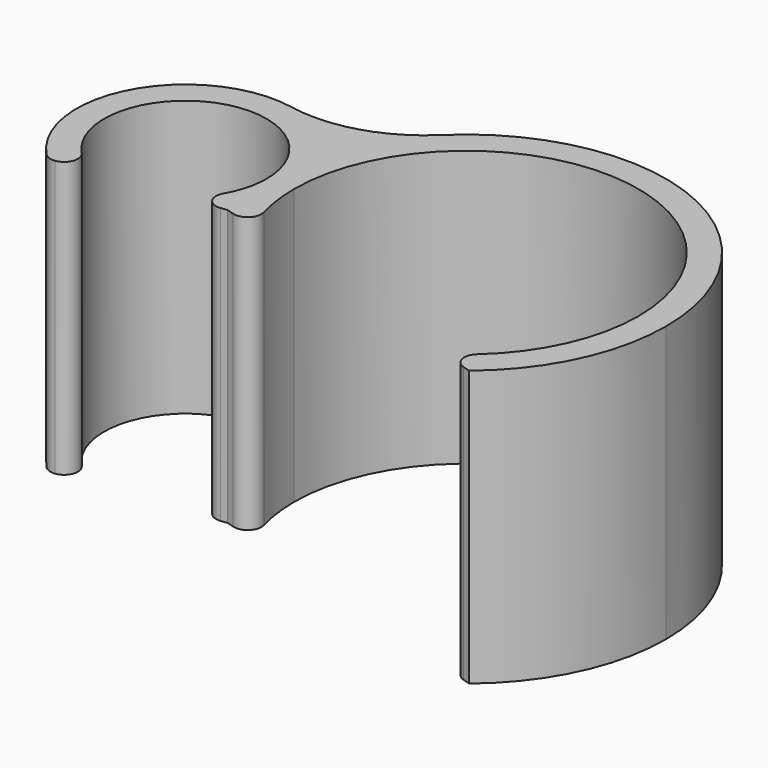
from build123d import *

# Parameters (mm, degrees)
F1_DEPTH = 10
F2_R     = 5
F3_R     = 0.49999


# Not quite as in the source:
# - a fillet or chamfer is up to 0.001 mm smaller than in the source, because OpenCascade refuses the exact size


with BuildPart() as f1:
    # F0 (on Top) → F1 (new body)
    with BuildSketch(Plane.XY):
        with BuildLine():
            ThreePointArc((-1.1283685941, -2.7256713514), (-1.6391785515, 2.4526707232), (2.95, 0))
            ThreePointArc((2.95, 0), (3.035057777, 1.107295327), (3.2882352941, 2.1886088391))
            ThreePointArc((3.2882352941, 2.1886088391), (-2.5695330315, 3), (-2.6678904245, -2.9128784188))
            Line((-2.6678904245, -2.9128784188), (-1.1283685941, -2.7256713514))
        make_face()
        with BuildLine():
            ThreePointArc((3.2882352941, 2.1886088391), (3.035057777, 1.107295327), (2.95, 0))
            ThreePointArc((2.95, 0), (3.035057777, -1.107295327), (3.2882352941, -2.1886088391))
            ThreePointArc((3.2882352941, -2.1886088391), (3.7809409815, -1.1432345753), (3.95, 0))
            ThreePointArc((3.95, 0), (3.7809409815, 1.1432345753), (3.2882352941, 2.1886088391))
        make_face()
        with BuildLine():
            ThreePointArc((3.2882352941, -2.1886088391), (3.035057777, -1.107295327), (2.95, 0))
            ThreePointArc((2.95, 0), (2.6326037224, -1.3311264557), (1.7487134637, -2.3758159065))
            Line((1.7487134637, -2.3758159065), (3.2882352941, -2.1886088391))
        make_face()
        with BuildLine():
            ThreePointArc((3.95, 0), (3.7809409815, -1.1432345753), (3.2882352941, -2.1886088391))
            Line((3.2882352941, -2.1886088391), (4.4925851142, -2.5471386536))
            ThreePointArc((4.4925851142, -2.5471386536), (4.0871511128, -1.3021438023), (3.95, 0))
        make_face()
        with BuildLine():
            ThreePointArc((17.45, 0), (11.307295327, 7.164942223), (3.2882352941, 2.1886088391))
            ThreePointArc((3.2882352941, 2.1886088391), (3.7809409815, 1.1432345753), (3.95, 0))
            ThreePointArc((3.95, 0), (10.2, 6.25), (16.45, 0))
            ThreePointArc((16.45, 0), (15.6872207282, -2.9921411532), (13.5850692222, -5.2539324663))
            Line((13.5850692222, -5.2539324663), (14.7894190423, -5.6124622809))
            ThreePointArc((14.7894190423, -5.6124622809), (16.7511750113, -3.1055765925), (17.45, 0))
        make_face()
    extrude(amount=F1_DEPTH)

    # F2
    f2_edges = [f1.edges().sort_by_distance(p)[0] for p in [
        (3.288235, 2.188609, 5),
    ]]
    fillet(f2_edges, radius=F2_R)

    # F3 (radius 0.5 in the source; OpenCascade refuses exactly that, so slightly less here)
    f3_edges = [f1.edges().sort_by_distance(p)[0] for p in [
        (-1.128369, -2.725671, 5),
        (1.748713, -2.375816, 5),
        (4.492585, -2.547139, 5),
        (13.585069, -5.253932, 5),
        (-2.66789, -2.912878, 5),
    ]]
    fillet(f3_edges, radius=F3_R)


solid = f1.part
